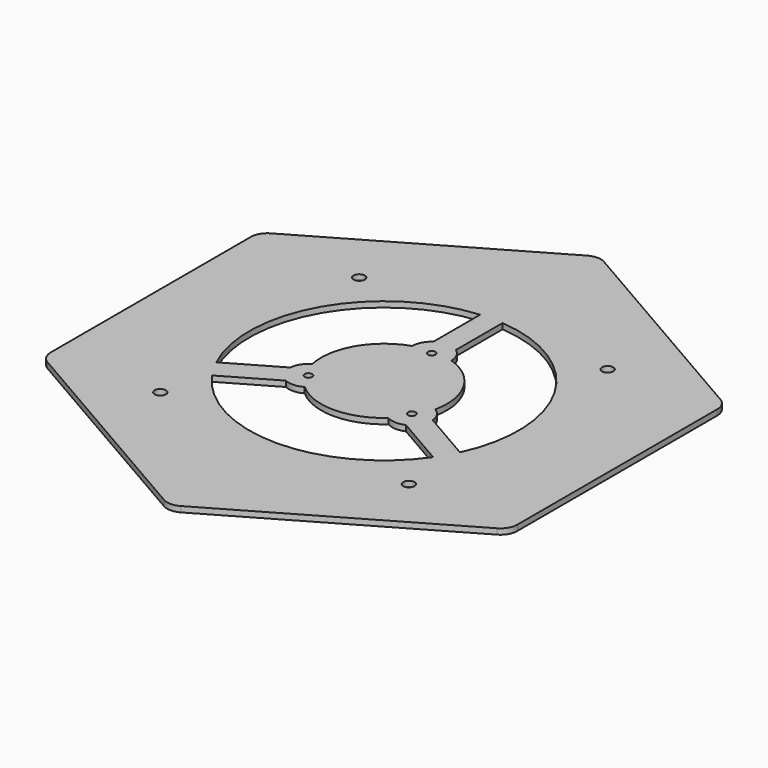
from build123d import *

# Parameters (mm, degrees)
F0_R            = 1.5875
F1_DEPTH        = 1.5875
F2_R            = 1.0922
F3_DEPTH        = 1.5875
F3_COPIES_COUNT = 3
F4_R            = 4.7625


# Not quite as in the source:
# - a pattern or mirror of a feature is missing from the dataset's text; its kind, count and spacing are read off the source's solid


with BuildPart() as f1:
    # F0 (on Top) → F1 (new body)
    with BuildSketch(Plane.XY):
        Polygon((65.9911357684, -38.1), (65.9911357684, 38.1), (0, 76.2), (-65.9911357684, 38.1), (-65.9911357684, -38.1), (0, -76.2), align=None)
        with Locations((-35.1536, -35.1536)):
            Circle(F0_R, mode=Mode.SUBTRACT)
        with Locations((35.1536, -35.1536)):
            Circle(F0_R, mode=Mode.SUBTRACT)
        with Locations((-35.1536, 35.1536)):
            Circle(F0_R, mode=Mode.SUBTRACT)
        with Locations((35.1536, 35.1536)):
            Circle(F0_R, mode=Mode.SUBTRACT)
    extrude(amount=F1_DEPTH)

    # F2 (on face) → F3 (cut, through all)
    with BuildSketch(Plane.XY.offset(1.5875)):
        with BuildLine():
            ThreePointArc((11.8486437632, -13.2566225326), (0, -17.78), (-11.8486437632, -13.2566225326))
            ThreePointArc((-11.8486437632, -13.2566225326), (-14.3916795622, -13.9960432527), (-16.9881251543, -13.4742728402))
            Line((-16.9881251543, -13.4742728402), (-31.2933003438, -21.7333695867))
            ThreePointArc((-31.2933003438, -21.7333695867), (0, -38.1), (31.2933003438, -21.7333695867))
            Line((31.2933003438, -21.7333695867), (16.9881251543, -13.4742728402))
            ThreePointArc((16.9881251543, -13.4742728402), (14.3916795622, -13.9960432527), (11.8486437632, -13.2566225326))
        make_face()
        with Locations((14.6267687632, -8.4447688828)):
            Circle(F2_R)
        with Locations((-14.6267687632, -8.4447688828)):
            Circle(F2_R)
    f3 = extrude(amount=-F3_DEPTH, mode=Mode.SUBTRACT)

    # F3_copies: F3 ×3 about axis
    f3_copies_axis = Axis((0, 0, 0), (0, 0, 1))
    for i in range(1, F3_COPIES_COUNT):
        add(f3.rotate(f3_copies_axis, i * 360 / F3_COPIES_COUNT), mode=Mode.SUBTRACT)

    # F4
    f4_edges = [f1.edges().sort_by_distance(p)[0] for p in [
        (-65.991136, 38.1, 0.79375),
        (0, 76.2, 0.79375),
        (65.991136, 38.1, 0.79375),
        (65.991136, -38.1, 0.79375),
        (0, -76.2, 0.79375),
        (-65.991136, -38.1, 0.79375),
    ]]
    fillet(f4_edges, radius=F4_R)


solid = f1.part
